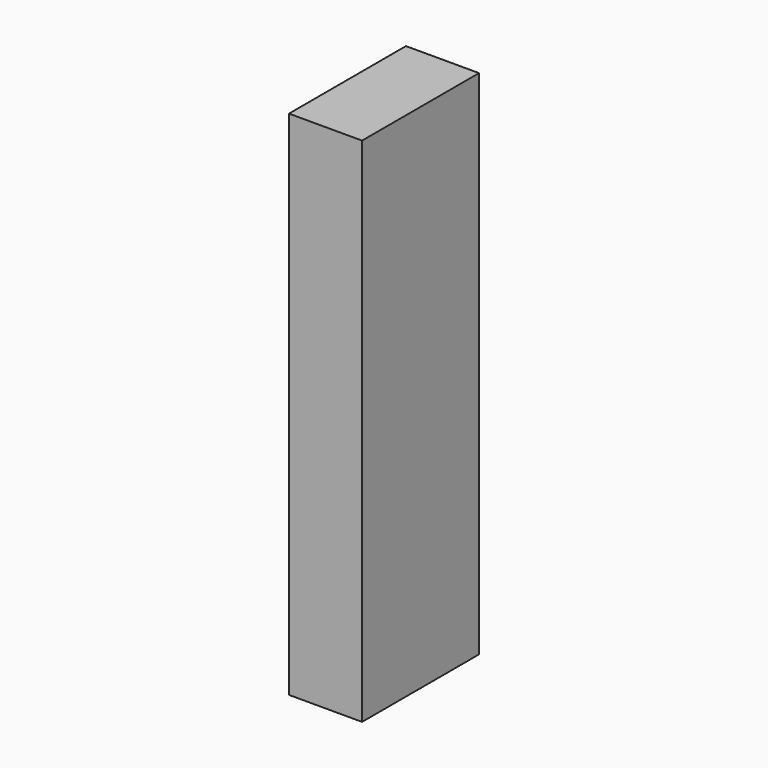
from build123d import *

# Parameters (mm, degrees)
F1_E0_W  = 311.15
F1_E0_H  = 88.9
F2_DEPTH = 44.45


with BuildPart() as f2:
    # F1_E0 (on explicit) → F2 (new body)
    with BuildSketch(Plane(origin=(-50.5113638937, 44.45, 153.1504544139), x_dir=(0, 0, -1), z_dir=(-1, 0, 0))):
        with Locations((155.575, 44.45)):
            Rectangle(F1_E0_W, F1_E0_H)
    extrude(amount=F2_DEPTH)


solid = f2.part
